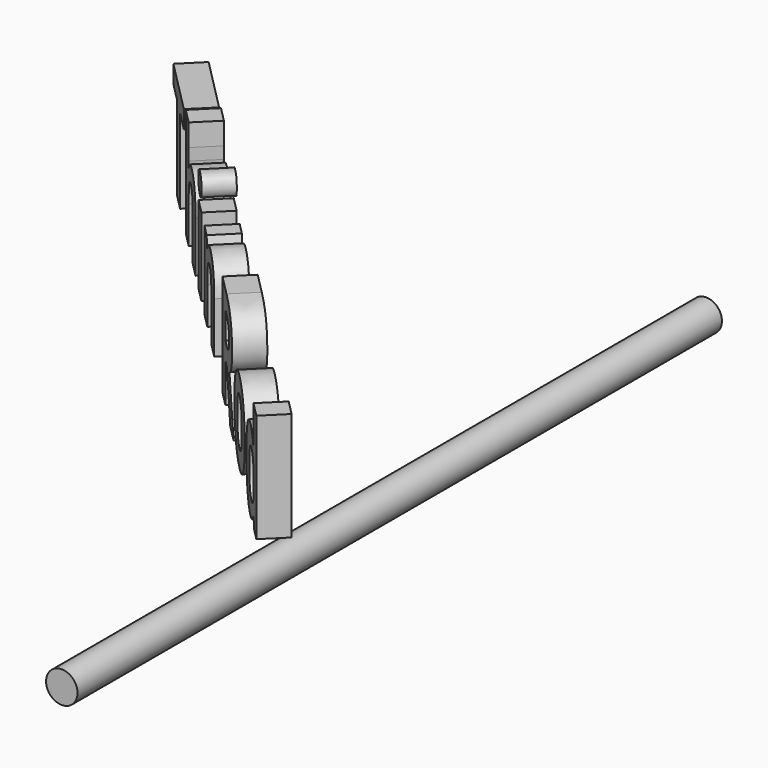
from build123d import *

# Parameters (mm, degrees)
F0_R          = 14.4488838609
F1_DEPTH      = 386.08
F1_DEPTH_BACK = 353.06
F4_TEXT_SIZE  = 131.2749253379
F5_DEPTH      = 25.4


# Not quite as in the source:
# - Text() gives the source's letters only with a copy of the font that has no kerning and outlines rounded to 1/6400 em; it was checked with that copy


with BuildPart() as f1:
    # F0 (on Front) → F1 (new body, two sides)
    with BuildSketch(Plane.XZ) as f1_sk:
        Circle(F0_R)
    extrude(amount=F1_DEPTH)
    extrude(f1_sk.sketch, amount=-F1_DEPTH_BACK)


with BuildPart() as f5:
    # F4 (on line) → F5 (new body)
    with BuildSketch(Plane(origin=(-79.0281668305, -78.3170908689, 0), x_dir=(0.7039040305, -0.7102950906, 0), z_dir=(-0.7102950906, -0.7039040305, 0))):
        with Locations((-241.6170015931, 136.7686986923)):
            Text('Thin Rod', F4_TEXT_SIZE, font='Open Sans', font_style=FontStyle.BOLD, text_align=(TextAlign.LEFT, TextAlign.BOTTOM))
    extrude(amount=F5_DEPTH)


solid = Compound([f1.part, f5.part])
